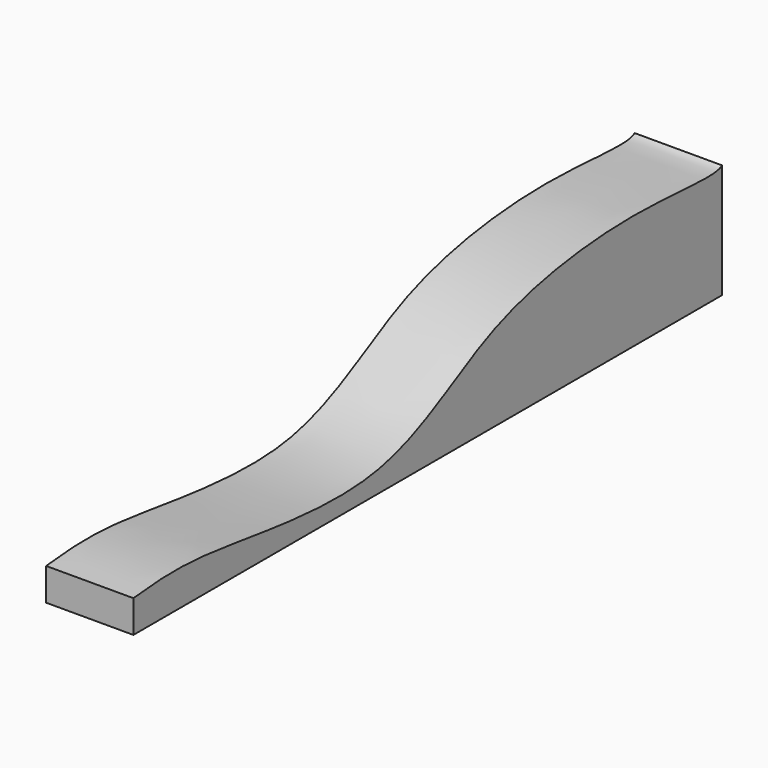
from build123d import *

# Parameters (mm, degrees)
F1_DEPTH = 30
F3_D     = 15
F3_DEPTH = 12
F3_TIP   = 4.5064546427


with BuildPart() as f1:
    # F0 (on Right) → F1 (new body)
    with BuildSketch(Plane.YZ):
        with BuildLine():
            add(Edge.make_bspline(
                [(-131.7461282015, -6.3447873108), (-123.3728835246, -5.5048995417), (-101.6398772811, -3.324945792), (-23.878808121, -20.0188151505), (17.9272379867, 14.4389849512), (65.4591264475, 22.4432346678), (95.6973111303, 22.0628570773), (119.1290489196, 19.9651290611), (120.9872886539, 21.8335315585)],
                knots=[0, 0, 0, 0, 0.0724770959, 0.1881164636, 0.2848952315, 0.3749576445, 0.4526977925, 0.5148099141, 0.5148099141, 0.5148099141, 0.5148099141], degree=3))
            Line((-131.7461282015, -6.3447873108), (-131.7461282015, -17.4702424556))
            Line((-131.7461282015, -17.4702424556), (120.9872886539, -17.4702424556))
            Line((120.9872886539, -17.4702424556), (120.9872886539, 21.8335315585))
        make_face()
    extrude(amount=F1_DEPTH)

    # F3
    with Locations(Plane(origin=(0, 120.9872886539, 0), x_dir=(-1, 0, 0), z_dir=(0, 1, 0))):
        with Locations((-16.6236571968, 0)):
            Hole(F3_D / 2, depth=F3_DEPTH)
            with Locations((0, 0, -(F3_DEPTH + F3_TIP / 2))):  # 118° drill point
                Cone(0, F3_D / 2, F3_TIP, mode=Mode.SUBTRACT)


solid = f1.part
